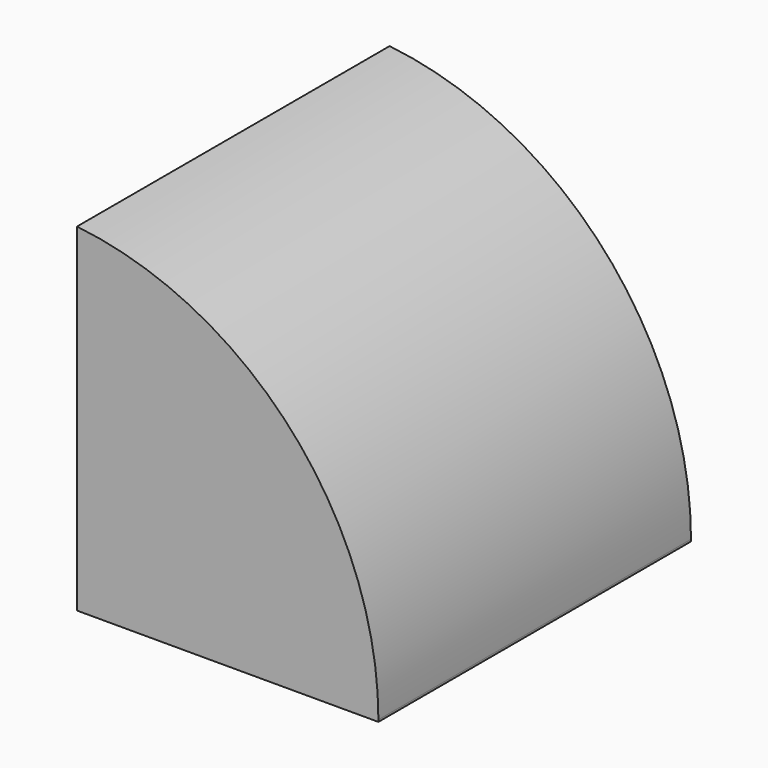
from build123d import *

# Parameters (mm, degrees)
F0_W        = 67.9279565811
F0_H        = 88.0647003651
F1_DEPTH    = 76.2
F2_T1_DEPTH = 466.8130765225


# Not quite as in the source:
# - a fillet or chamfer that OpenCascade refuses, or shapes differently, is made with other operations: its cross-section is extruded or revolved along the edge and cut away or added


with BuildPart() as f1:
    # F0 (on Top) → F1 (new body)
    with BuildSketch(Plane.XY):
        Rectangle(F0_W, F0_H)
    extrude(amount=F1_DEPTH)

    # F2: fillet of radius 76.2 on 1 edges, made by hand

    # F2_s2 → F2_t1 (cut)
    with BuildSketch(Plane.XZ.offset(-233.4065382613)):
        with BuildLine():
            ThreePointArc((33.9639782906, 0.4503247685), (14.4947887401, 51.3232561342), (-33.9639782906, 76.2))
            Line((-33.9639782906, 76.2), (33.9639782906, 76.2))
            Line((33.9639782906, 76.2), (33.9639782906, 0.4503247685))
        make_face()
    extrude(amount=F2_T1_DEPTH, mode=Mode.SUBTRACT)


solid = f1.part
